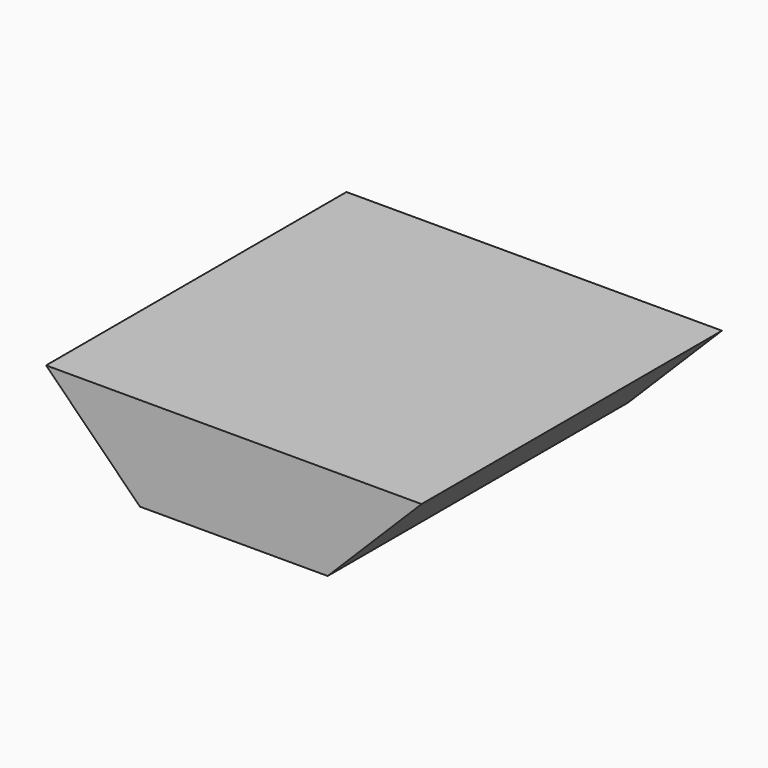
from build123d import *

# Parameters (mm, degrees)
F0_W     = 100
F0_H     = 100
F1_DEPTH = 25
F2_SIZE  = 24.99999


# Not quite as in the source:
# - a fillet or chamfer is up to 0.001 mm smaller than in the source, because OpenCascade refuses the exact size


with BuildPart() as f1:
    # F0 (on Top) → F1 (new body)
    with BuildSketch(Plane.XY):
        Rectangle(F0_W, F0_H)
    extrude(amount=F1_DEPTH)

    # F2 (size 25 in the source; OpenCascade refuses exactly that, so slightly less here)
    f2_edges = [f1.edges().sort_by_distance(p)[0] for p in [
        (50, 0, 0),
        (-50, 0, 0),
    ]]
    chamfer(f2_edges, length=F2_SIZE)


solid = f1.part
